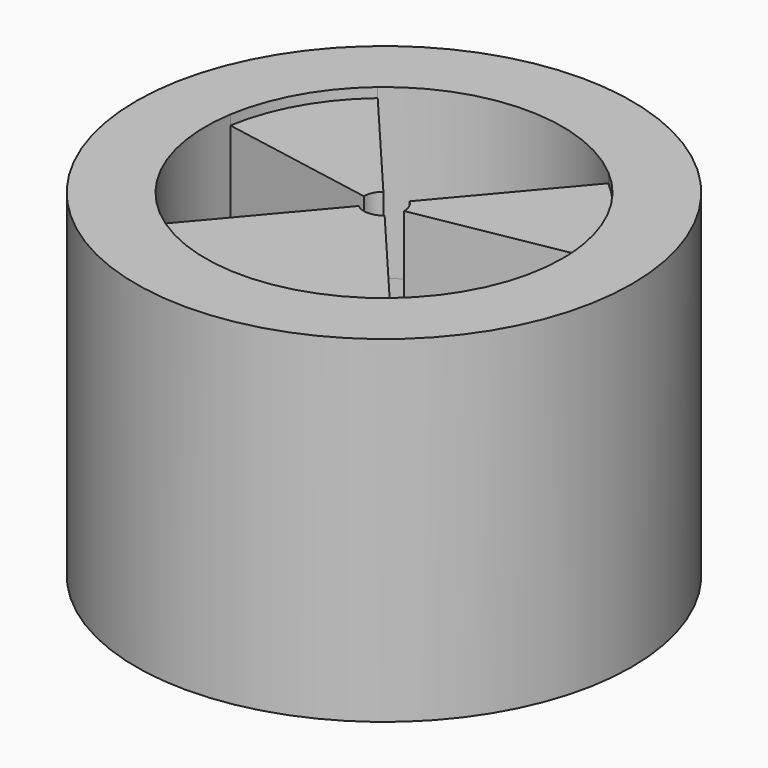
from build123d import *

# Parameters (mm, degrees)
F0_R     = 7.0954565199
F1_DEPTH = 4.826
F2_DEPTH = 4.5466


# Not quite as in the source:
# - the program builds the solid bodies; features that only make, move or delete a surface that nothing else refers to are left out


with BuildPart() as f1:
    # F0 (on Top) → F1 (new body, symmetric)
    with BuildSketch(Plane.XY):
        Circle(F0_R)
        with BuildLine():
            ThreePointArc((3.3010527039, 3.9012801832), (4.4504568739, 2.5120449112), (5.045856518, 0.8101037104))
            ThreePointArc((5.045856518, 0.8101037104), (5.0942933944, 0.4063383238), (5.1104731701, 0))
            ThreePointArc((5.1104731701, 0), (4.6361016651, -2.1502319347), (3.3010527039, -3.9012801832))
            ThreePointArc((3.3010527039, -3.9012801832), (0, -5.1104731701), (-3.3010527039, -3.9012801832))
            ThreePointArc((-3.3010527039, -3.9012801832), (-4.7923906287, -1.7748036747), (-5.045856518, 0.8101037104))
            ThreePointArc((-5.045856518, 0.8101037104), (-4.4504568739, 2.5120449112), (-3.3010527039, 3.9012801832))
            ThreePointArc((-3.3010527039, 3.9012801832), (0, 5.1104731701), (3.3010527039, 3.9012801832))
        make_face(mode=Mode.SUBTRACT)
    extrude(amount=F1_DEPTH, both=True)

    # F0 (on Top) → F2 (join, symmetric)
    with BuildSketch(Plane.XY):
        with BuildLine():
            ThreePointArc((0.3718910489, 0.4422755592), (0.5238357878, 0.243939931), (0.57785, 0))
            Line((0.57785, 0), (5.045856518, 0.8101037104))
            ThreePointArc((5.045856518, 0.8101037104), (4.4504568739, 2.5120449112), (3.3010527039, 3.9012801832))
            Line((3.3010527039, 3.9012801832), (0.3718910489, 0.4422755592))
        make_face()
        with BuildLine():
            ThreePointArc((-0.57785, 0), (-0.5238357878, 0.243939931), (-0.3718910489, 0.4422755592))
            Line((-0.3718910489, 0.4422755592), (-3.3010527039, 3.9012801832))
            ThreePointArc((-3.3010527039, 3.9012801832), (-4.4504568739, 2.5120449112), (-5.045856518, 0.8101037104))
            Line((-5.045856518, 0.8101037104), (-0.57785, 0))
        make_face()
        with BuildLine():
            Line((3.3010527039, -3.9012801832), (0.3718910489, -0.4422755592))
            ThreePointArc((0.3718910489, -0.4422755592), (0, -0.57785), (-0.3718910489, -0.4422755592))
            Line((-0.3718910489, -0.4422755592), (-3.3010527039, -3.9012801832))
            ThreePointArc((-3.3010527039, -3.9012801832), (0, -5.1104731701), (3.3010527039, -3.9012801832))
        make_face()
    extrude(amount=F2_DEPTH, both=True)


solid = f1.part
